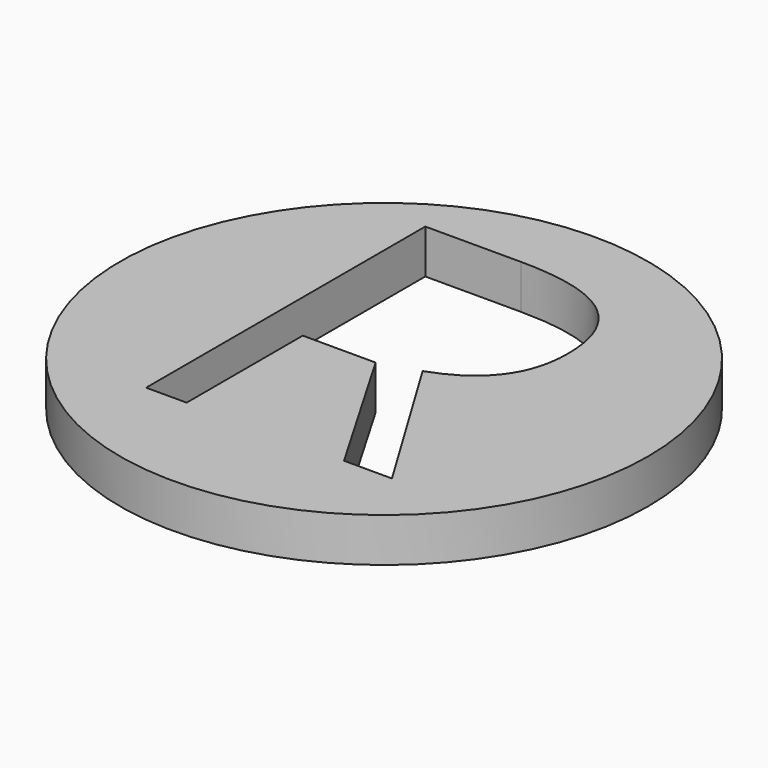
from build123d import *

# Parameters (mm, degrees)
F0_R         = 12
F1_DEPTH     = 2
F2_TEXT_SIZE = 22.2222222222
F3_DEPTH     = 25


# Not quite as in the source:
# - Text() gives the source's letters only with a copy of the font that has no kerning and outlines rounded to 1/6400 em; it was checked with that copy


with BuildPart() as f1:
    # F0 (on Top) → F1 (new body)
    with BuildSketch(Plane.XY):
        Circle(F0_R)
    extrude(amount=F1_DEPTH)

    # F2 (on face) → F3 (cut)
    with BuildSketch(Plane.XY.offset(2)):
        with Locations((-7.3993055556, -7)):
            Text('R', F2_TEXT_SIZE, font='Open Sans', text_align=(TextAlign.LEFT, TextAlign.BOTTOM))
        with BuildLine():
            Line((-3.375, 7.2465277778), (-3.375, 1.1805555556))
            Line((-3.375, 1.1805555556), (-0.84375, 1.1805555556))
            add(Edge.make_bspline(
                [(-0.84375, 1.1805555556), (1.1076388889, 1.1805555556), (2.0190972222, 1.9565972222)],
                knots=[0, 0, 0, 1, 1, 1], degree=2))
            add(Edge.make_bspline(
                [(2.0190972222, 1.9565972222), (2.9305555556, 2.7326388889), (2.9305555556, 4.2847222222)],
                knots=[0, 0, 0, 1, 1, 1], degree=2))
            add(Edge.make_bspline(
                [(2.9305555556, 4.2847222222), (2.9305555556, 5.8576388889), (2.0034722222, 6.5520833333)],
                knots=[0, 0, 0, 1, 1, 1], degree=2))
            add(Edge.make_bspline(
                [(2.0034722222, 6.5520833333), (1.0763888889, 7.2465277778), (-0.9756944444, 7.2465277778)],
                knots=[0, 0, 0, 1, 1, 1], degree=2))
            Line((-0.9756944444, 7.2465277778), (-3.375, 7.2465277778))
        make_face()
    extrude(amount=-F3_DEPTH, mode=Mode.SUBTRACT)


solid = f1.part
